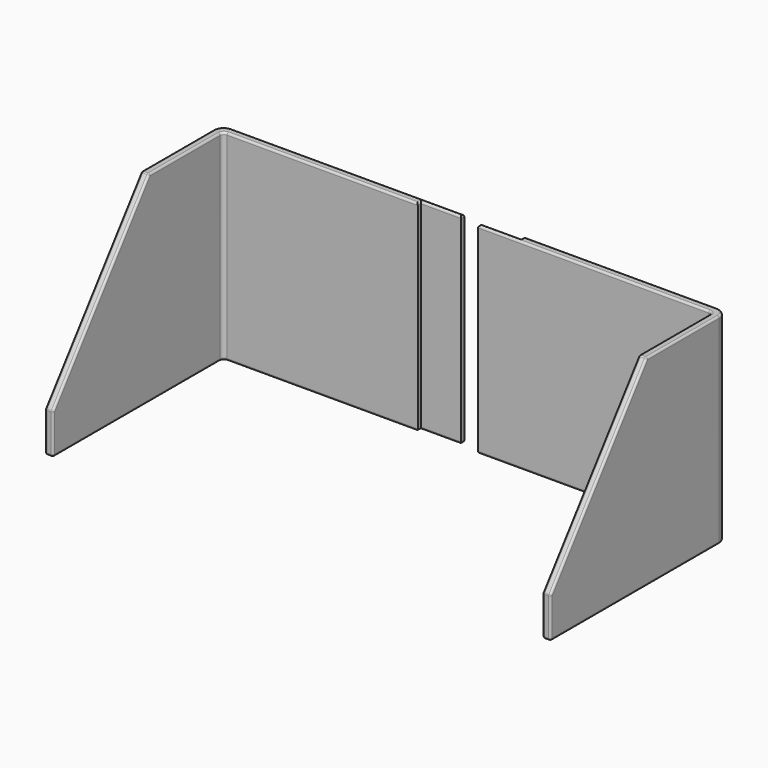
from build123d import *

# Parameters (mm, degrees)
F1_DEPTH = 100
F2_DEPTH = 100
F4_DEPTH = 25
F6_DEPTH = 25
F7_R     = 5
F7_2_R   = 5
F8_R     = 2
F8_2_R   = 2
F9_R     = 0.99999
F9_2_R   = 0.99999


# Not quite as in the source:
# - a fillet or chamfer is up to 0.001 mm smaller than in the source, because OpenCascade refuses the exact size


with BuildPart() as f1:
    # F0 (on Top) → F1 (new body)
    with BuildSketch(Plane.XY):
        Polygon((107, 0), (10, 0), (10, -2), (-10, -2), (-10, -4), (107, -4), (107, -110), (111, -110), (111, 0), align=None)
    extrude(amount=F1_DEPTH)

    # F3 (on face) → F4 (cut)
    with BuildSketch(Plane.YZ.offset(111)):
        Polygon((-110, 20), (-50, 100), (-110, 100), align=None)
    extrude(amount=-F4_DEPTH, mode=Mode.SUBTRACT)

    # F7
    f7_edges = [f1.edges().sort_by_distance(p)[0] for p in [
        (111, 0, 50),
    ]]
    fillet(f7_edges, radius=F7_R)

    # F8#2
    f8_2_edges = [f1.edges().sort_by_distance(p)[0] for p in [
        (107, -4, 50),
    ]]
    fillet(f8_2_edges, radius=F8_2_R)

    # F9#2 (radius 1 in the source; OpenCascade refuses exactly that, so slightly less here)
    f9_2_edges = [f1.edges().sort_by_distance(p)[0] for p in [
        (107, -28, 100),
        (106.414214, -4.585786, 100),
        (109, -50, 100),
        (47.5, -4, 100),
        (111, -27.5, 100),
        (-10, -3, 100),
        (109.535534, -1.464466, 100),
        (0, -2, 100),
        (58, 0, 100),
        (10, -1, 100),
        (111, -80, 60),
        (107, -80, 60),
        (109, -110, 20),
        (107, -58, 0),
        (106.414214, -4.585786, 0),
        (109, -110, 0),
        (47.5, -4, 0),
        (111, -57.5, 0),
        (-10, -3, 0),
        (109.535534, -1.464466, 0),
        (0, -2, 0),
        (58, 0, 0),
        (10, -1, 0),
        (111, -110, 10),
        (107, -110, 10),
    ]]
    fillet(f9_2_edges, radius=F9_2_R)


with BuildPart() as f2:
    # F0 (on Top) → F2 (new body)
    with BuildSketch(Plane.XY):
        Polygon((-20.0161703825, 0), (-141.0161703825, 0), (-141.0161703825, -110), (-137.0161703825, -110), (-137.0161703825, -4), (-40.0161703825, -4), (-40.0161703825, -2), (-20.0161703825, -2), align=None)
    extrude(amount=F2_DEPTH)

    # F5 (on face) → F6 (cut)
    with BuildSketch(Plane(origin=(-141.0161703825, 0, 0), x_dir=(0, -1, 0), z_dir=(-1, 0, 0))):
        Polygon((110, 100), (50, 100), (110, 20), align=None)
    extrude(amount=-F6_DEPTH, mode=Mode.SUBTRACT)

    # F7#2
    f7_2_edges = [f2.edges().sort_by_distance(p)[0] for p in [
        (-141.01617, 0, 50),
    ]]
    fillet(f7_2_edges, radius=F7_2_R)

    # F8
    f8_edges = [f2.edges().sort_by_distance(p)[0] for p in [
        (-137.01617, -4, 50),
    ]]
    fillet(f8_edges, radius=F8_R)

    # F9 (radius 1 in the source; OpenCascade refuses exactly that, so slightly less here)
    f9_edges = [f2.edges().sort_by_distance(p)[0] for p in [
        (-137.01617, -28, 100),
        (-136.430384, -4.585786, 100),
        (-139.01617, -50, 100),
        (-87.51617, -4, 100),
        (-141.01617, -27.5, 100),
        (-40.01617, -3, 100),
        (-139.551704, -1.464466, 100),
        (-30.01617, -2, 100),
        (-78.01617, 0, 100),
        (-20.01617, -1, 100),
        (-141.01617, -80, 60),
        (-139.01617, -110, 20),
        (-137.01617, -80, 60),
        (-137.01617, -58, 0),
        (-136.430384, -4.585786, 0),
        (-139.01617, -110, 0),
        (-87.51617, -4, 0),
        (-141.01617, -57.5, 0),
        (-40.01617, -3, 0),
        (-139.551704, -1.464466, 0),
        (-30.01617, -2, 0),
        (-78.01617, 0, 0),
        (-20.01617, -1, 0),
        (-137.01617, -110, 10),
        (-141.01617, -110, 10),
    ]]
    fillet(f9_edges, radius=F9_R)


solid = Compound([f1.part, f2.part])
